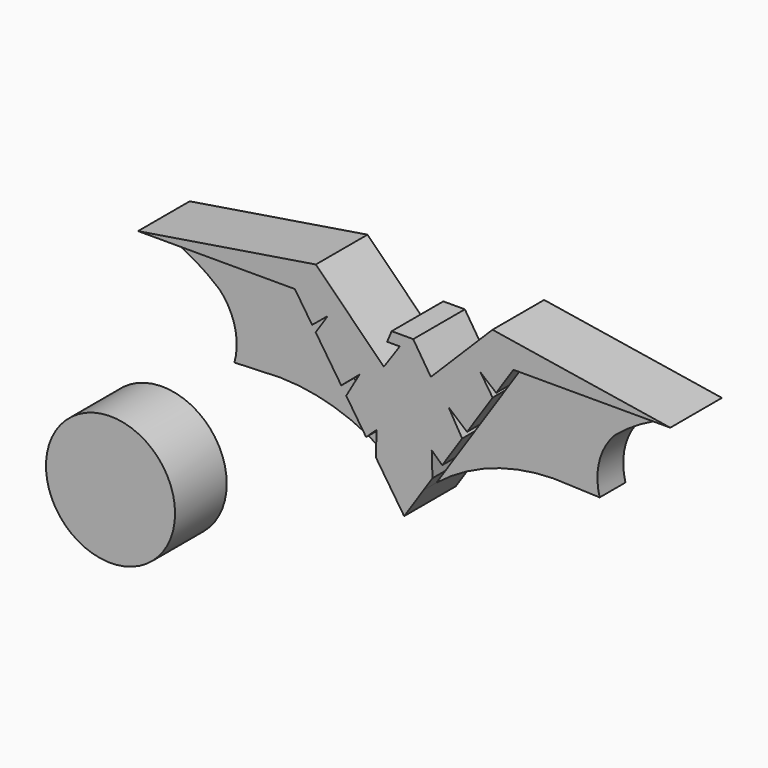
from build123d import *

# Parameters (mm, degrees)
F1_DEPTH = 6.35
F2_DEPTH = 3.175
F3_R     = 12.7
F4_DEPTH = 12.7


# Not quite as in the source:
# - a feature names something its author has since deleted; it is built from what else it names


with BuildPart() as f1:
    # F0 (on Front) → F1 (new body, symmetric)
    with BuildSketch(Plane.XZ):
        Polygon((1.7863946268, 11.7875747383), (0, 11.7875747383), (-2.4559120648, 11.7875747383), (-3.3509915229, 9.6617611125), (-0.8608896751, 9.6617611125), (-4.0002167225, 5.1155993715), (-17.3656828701, 18.4895154089), (-52.352450788, 12.8932353109), (-21.4979629964, 12.8932353109), (-18.104581877, 7.788236776), (-15.0197930634, 10.3294737637), (-17.406011636, 6.7373085332), (-12.3725614796, -0.8350079177), (-8.7693203241, 2.2335082758), (-11.3994373246, -2.2989747433), (-7.4821490115, -8.1921386397), (-5.4247728549, -6.2737190165), (-5.5697021181, -11.06922148), (-3.8242271729, -13.6951119192), (0, -19.4482747465), (3.8242271729, -13.6951119192), (5.5697021181, -11.06922148), (5.4247728549, -6.2737190165), (7.4821490115, -8.1921386397), (11.3994373246, -2.2989747433), (8.7693203241, 2.2335082758), (12.3725614796, -0.8350079177), (17.406011636, 6.7373085332), (15.0197930634, 10.3294737637), (18.104581877, 7.788236776), (21.4979629964, 12.8932353109), (52.352450788, 12.8932353109), (17.3786748844, 18.4874372818), (5.2548269741, 6.3712494448), align=None)
    extrude(amount=F1_DEPTH, both=True)

    # F0 (on Front) → F2 (join, symmetric)
    with BuildSketch(Plane.XZ):
        Polygon((1.7863946268, 11.7875747383), (0, 11.7875747383), (-2.4559120648, 11.7875747383), (-3.3509915229, 9.6617611125), (-0.8608896751, 9.6617611125), (-4.0002167225, 5.1155993715), (-17.3656828701, 18.4895154089), (-52.352450788, 12.8932353109), (-21.4979629964, 12.8932353109), (-18.104581877, 7.788236776), (-15.0197930634, 10.3294737637), (-17.406011636, 6.7373085332), (-12.3725614796, -0.8350079177), (-8.7693203241, 2.2335082758), (-11.3994373246, -2.2989747433), (-7.4821490115, -8.1921386397), (-5.4247728549, -6.2737190165), (-5.5697021181, -11.06922148), (-3.8242271729, -13.6951119192), (0, -19.4482747465), (3.8242271729, -13.6951119192), (5.5697021181, -11.06922148), (5.4247728549, -6.2737190165), (7.4821490115, -8.1921386397), (11.3994373246, -2.2989747433), (8.7693203241, 2.2335082758), (12.3725614796, -0.8350079177), (17.406011636, 6.7373085332), (15.0197930634, 10.3294737637), (18.104581877, 7.788236776), (21.4979629964, 12.8932353109), (52.352450788, 12.8932353109), (17.3786748844, 18.4874372818), (5.2548269741, 6.3712494448), align=None)
        with BuildLine():
            ThreePointArc((38.8560444117, 5.8900536969), (45.2033351378, 10.1642758317), (52.352450788, 12.8932353109))
            Line((52.352450788, 12.8932353109), (21.4979629964, 12.8932353109))
            Line((21.4979629964, 12.8932353109), (18.104581877, 7.788236776))
            Line((18.104581877, 7.788236776), (17.406011636, 6.7373085332))
            Line((17.406011636, 6.7373085332), (12.3725614796, -0.8350079177))
            Line((12.3725614796, -0.8350079177), (11.3994373246, -2.2989747433))
            Line((11.3994373246, -2.2989747433), (7.4821490115, -8.1921386397))
            Line((7.4821490115, -8.1921386397), (5.5697021181, -11.06922148))
            Line((5.5697021181, -11.06922148), (3.8242271729, -13.6951119192))
            ThreePointArc((3.8242271729, -13.6951119192), (16.3311358391, -7.118704323), (30.380692333, -5.6081204675))
            Line((30.380692333, -5.6081204675), (35.918712616, -5.8190925047))
            ThreePointArc((35.918712616, -5.8190925047), (35.8448269076, 0.4224418486), (38.8560444117, 5.8900536969))
        make_face()
        with BuildLine():
            Line((-21.4979629964, 12.8932353109), (-52.352450788, 12.8932353109))
            ThreePointArc((-52.352450788, 12.8932353109), (-45.2033351378, 10.1642758317), (-38.8560444117, 5.8900536969))
            ThreePointArc((-38.8560444117, 5.8900536969), (-35.8448269076, 0.4224418486), (-35.918712616, -5.8190925047))
            Line((-35.918712616, -5.8190925047), (-30.380692333, -5.6081204675))
            ThreePointArc((-30.380692333, -5.6081204675), (-16.3311358391, -7.118704323), (-3.8242271729, -13.6951119192))
            Line((-3.8242271729, -13.6951119192), (-5.5697021181, -11.06922148))
            Line((-5.5697021181, -11.06922148), (-7.4821490115, -8.1921386397))
            Line((-7.4821490115, -8.1921386397), (-11.3994373246, -2.2989747433))
            Line((-11.3994373246, -2.2989747433), (-12.3725614796, -0.8350079177))
            Line((-12.3725614796, -0.8350079177), (-17.406011636, 6.7373085332))
            Line((-17.406011636, 6.7373085332), (-18.104581877, 7.788236776))
            Line((-18.104581877, 7.788236776), (-21.4979629964, 12.8932353109))
        make_face()
    extrude(amount=F2_DEPTH, both=True)


with BuildPart() as f4:
    # F3 (on Front) → F4 (new body)
    with BuildSketch(Plane.XZ):
        with Locations((-52.6836439967, -29.408633709)):
            Circle(F3_R)
    extrude(amount=F4_DEPTH)


solid = Compound([f1.part, f4.part])
